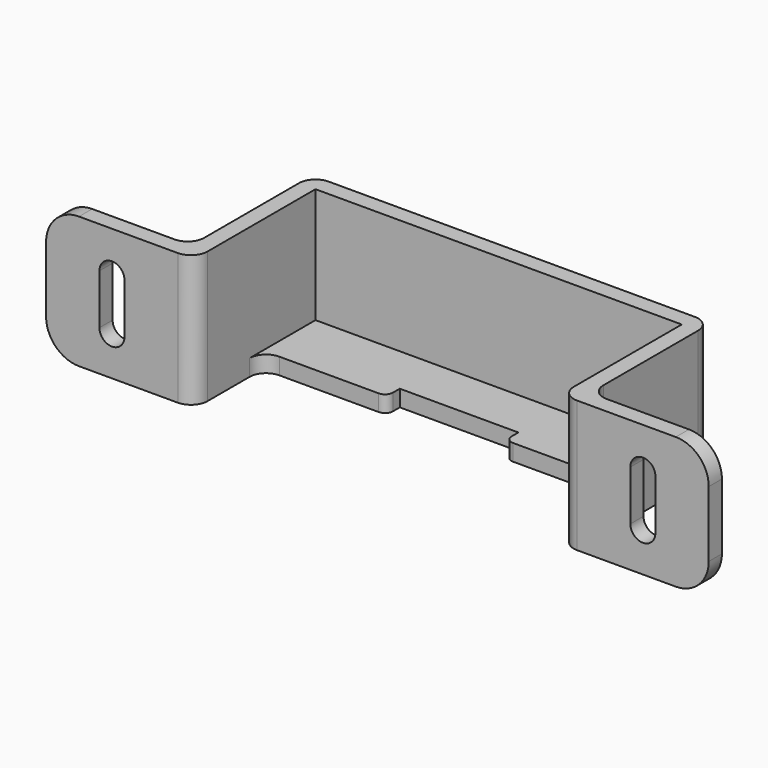
from build123d import *

# Parameters (mm, degrees)
F1_DEPTH  = 25.4
F2_R      = 3.175
F4_DEPTH  = 32.386
F5_R      = 6.35
F6_W      = 70.612
F6_H      = 12.7
F7_DEPTH  = 3.175
F8_R      = 3.175
F9_W      = 22.86
F9_H      = 3.175
F10_DEPTH = 25.4
F11_R     = 1.524


with BuildPart() as f1:
    # F0 (on Top) → F1 (new body)
    with BuildSketch(Plane.XY):
        Polygon((-35.306, 29.21), (0, 29.21), (35.306, 29.21), (35.306, 0), (63.881, 0), (63.881, 3.175), (38.481, 3.175), (38.481, 32.385), (0, 32.385), (-38.481, 32.385), (-38.481, 3.175), (-63.881, 3.175), (-63.881, 0), (-35.306, 0), align=None)
    extrude(amount=F1_DEPTH)

    # F2
    f2_edges = [f1.edges().sort_by_distance(p)[0] for p in [
        (-35.306, 0, 12.7),
        (35.306, 0, 12.7),
    ]]
    fillet(f2_edges, radius=F2_R)

    # F3 (on Front) → F4 (cut, through all)
    with BuildSketch(Plane.XZ):
        with BuildLine():
            ThreePointArc((-53.594, 7.8105), (-51.181, 5.3975), (-48.768, 7.8105))
            Line((-48.768, 7.8105), (-48.768, 17.4625))
            ThreePointArc((-48.768, 17.4625), (-51.181, 19.8755), (-53.594, 17.4625))
            Line((-53.594, 17.4625), (-53.594, 7.8105))
        make_face()
        with BuildLine():
            ThreePointArc((53.594, 17.4498), (51.181, 19.8628), (48.768, 17.4498))
            Line((48.768, 17.4498), (48.768, 7.7978))
            ThreePointArc((48.768, 7.7978), (51.181, 5.3848), (53.594, 7.7978))
            Line((53.594, 7.7978), (53.594, 17.4498))
        make_face()
    extrude(amount=-F4_DEPTH, mode=Mode.SUBTRACT)

    # F5
    f5_edges = [f1.edges().sort_by_distance(p)[0] for p in [
        (-63.881, 1.5875, 0),
        (-63.881, 1.5875, 25.4),
        (63.881, 1.5875, 25.4),
        (63.881, 1.5875, 0),
    ]]
    fillet(f5_edges, radius=F5_R)

    # F6 (on face) → F7 (join)
    with BuildSketch(Plane(origin=(0, 0, 0), x_dir=(1, 0, 0), z_dir=(0, 0, -1))):
        with Locations((0, -22.86)):
            Rectangle(F6_W, F6_H)
    extrude(amount=-F7_DEPTH)

    # F8
    f8_edges = [f1.edges().sort_by_distance(p)[0] for p in [
        (38.481, 3.175, 12.7),
        (38.481, 32.385, 12.7),
        (-38.481, 32.385, 12.7),
        (-38.481, 3.175, 12.7),
        (35.306, 16.51, 1.5875),
        (-35.306, 16.51, 1.5875),
    ]]
    fillet(f8_edges, radius=F8_R)

    # F9 (on face) → F10 (cut)
    with BuildSketch(Plane.XY.offset(3.175)):
        with Locations((0, 18.0975)):
            Rectangle(F9_W, F9_H)
    extrude(amount=-F10_DEPTH, mode=Mode.SUBTRACT)

    # F11
    f11_edges = [f1.edges().sort_by_distance(p)[0] for p in [
        (-11.43, 16.51, 1.5875),
        (11.43, 16.51, 1.5875),
    ]]
    fillet(f11_edges, radius=F11_R)


solid = f1.part
